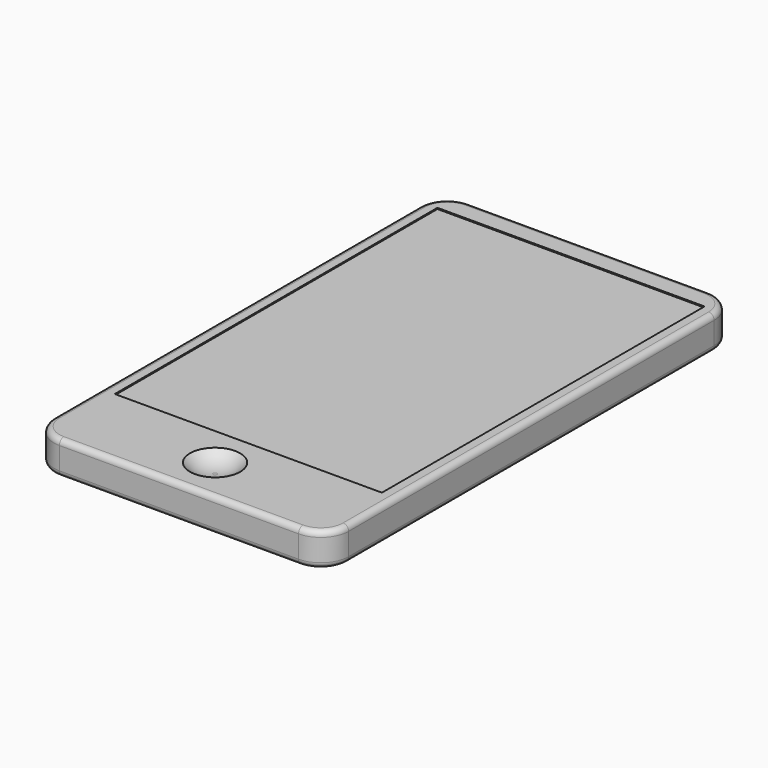
from build123d import *

# Parameters (mm, degrees)
F1_DEPTH  = 3.81
F2_R      = 1.27
F3_R      = 5.7323628205
F4_DEPTH  = 2.286
F3_W      = 60.96
F3_H      = 92.0373842978
F6_DEPTH  = 0.254
F7_W      = 12.1530219913
F7_H      = 2.4910259526
F8_DEPTH  = 1.1176
F9_R      = 0.9198153673
F11_DEPTH = 1.6002
F12_R     = 0.3066051224


# Not quite as in the source:
# - a fillet or chamfer that OpenCascade refuses, or shapes differently, is made with other operations: its cross-section is extruded or revolved along the edge and cut away or added


with BuildPart() as f1:
    # F0 (on Top) → F1 (new body, symmetric)
    with BuildSketch(Plane.XY):
        with BuildLine():
            Line((-27.2898482323, -58.4841631353), (27.2898482323, -58.4841631353))
            ThreePointArc((27.2898482323, -58.4841631353), (31.7799762928, -56.6242911958), (33.6398482323, -52.1341631353))
            Line((33.6398482323, -52.1341631353), (33.6398482323, 52.1341631353))
            ThreePointArc((33.6398482323, 52.1341631353), (31.7799762928, 56.6242911958), (27.2898482323, 58.4841631353))
            Line((27.2898482323, 58.4841631353), (-27.2898482323, 58.4841631353))
            ThreePointArc((-27.2898482323, 58.4841631353), (-31.7799762928, 56.6242911958), (-33.6398482323, 52.1341631353))
            Line((-33.6398482323, 52.1341631353), (-33.6398482323, -52.1341631353))
            ThreePointArc((-33.6398482323, -52.1341631353), (-31.7799762928, -56.6242911958), (-27.2898482323, -58.4841631353))
        make_face()
    extrude(amount=F1_DEPTH, both=True)

    # F2
    f2_edges = [f1.edges().sort_by_distance(p)[0] for p in [
        (33.639848, 0, 3.81),
        (33.639848, 0, -3.81),
        (-33.639848, 0, -3.81),
        (-33.639848, 0, 3.81),
        (-31.779976, 56.624291, -3.81),
        (-31.779976, 56.624291, 3.81),
        (0, 58.484163, -3.81),
        (0, 58.484163, 3.81),
        (31.779976, 56.624291, -3.81),
        (31.779976, 56.624291, 3.81),
        (31.779976, -56.624291, -3.81),
        (31.779976, -56.624291, 3.81),
        (0, -58.484163, -3.81),
        (0, -58.484163, 3.81),
        (-31.779976, -56.624291, 3.81),
        (-31.779976, -56.624291, -3.81),
    ]]
    fillet(f2_edges, radius=F2_R)

    # F3 (on face) → F4 (cut)
    with BuildSketch(Plane.XY.offset(3.81)):
        with Locations((0, -48.1907315552)):
            Circle(F3_R)
    extrude(amount=-F4_DEPTH, mode=Mode.SUBTRACT)

    # F5: fillet of radius 7.2972019136 on 1 edges, made by hand

    # F5_s1 → F5_t2 (revolve)
    with BuildSketch(Plane.XZ.offset(48.1907315552)):
        with BuildLine():
            ThreePointArc((5.7323628205, 3.81), (3.3159569781, 2.1198248924), (0.4279296605, 1.524))
            Line((0.4279296605, 1.524), (5.7323628205, 1.524))
            Line((5.7323628205, 1.524), (5.7323628205, 3.81))
        make_face()
    revolve(axis=Axis((0, -48.1907315552, 1.524), (0, 0, 1)))

    # F3 (on face) → F6 (cut)
    with BuildSketch(Plane.XY.offset(3.81)):
        with Locations((0, 7.3213078511)):
            Rectangle(F3_W, F3_H)
    extrude(amount=-F6_DEPTH, mode=Mode.SUBTRACT)

    # F7 (on face) → F8 (cut)
    with BuildSketch(Plane(origin=(-33.6398482323, 0, 0), x_dir=(0, -1, 0), z_dir=(-1, 0, 0))):
        with Locations((-43.15578565, 0)):
            Rectangle(F7_W, F7_H)
    extrude(amount=-F8_DEPTH, mode=Mode.SUBTRACT)

    # F9
    f9_edges = [f1.edges().sort_by_distance(p)[0] for p in [
        (-33.081048, 37.079275, 1.245513),
        (-33.081048, 49.232297, 1.245513),
        (-33.081048, 49.232297, -1.245513),
        (-33.081048, 37.079275, -1.245513),
    ]]
    fillet(f9_edges, radius=F9_R)


with BuildPart() as f11:
    # F10 (on face) → F11 (new body)
    with BuildSketch(Plane(origin=(-32.5222482323, 0, 0), x_dir=(0, -1, 0), z_dir=(-1, 0, 0))):
        with BuildLine():
            Line((-48.3124812784, -1.0677123209), (-37.9990900217, -1.0677123209))
            ThreePointArc((-37.9990900217, -1.0677123209), (-37.4744063871, -0.8503812436), (-37.2570753098, -0.325697609))
            Line((-37.2570753098, -0.325697609), (-37.2570753098, 0.325697609))
            ThreePointArc((-37.2570753098, 0.325697609), (-37.4744063871, 0.8503812436), (-37.9990900217, 1.0677123209))
            Line((-37.9990900217, 1.0677123209), (-48.3124812784, 1.0677123209))
            ThreePointArc((-48.3124812784, 1.0677123209), (-48.8371649129, 0.8503812436), (-49.0544959903, 0.325697609))
            Line((-49.0544959903, 0.325697609), (-49.0544959903, -0.325697609))
            ThreePointArc((-49.0544959903, -0.325697609), (-48.8371649129, -0.8503812436), (-48.3124812784, -1.0677123209))
        make_face()
    extrude(amount=F11_DEPTH)

    # F12
    f12_edges = [f11.edges().sort_by_distance(p)[0] for p in [
        (-34.122448, 37.474406, -0.850381),
        (-34.122448, 37.257075, 0),
        (-34.122448, 37.474406, 0.850381),
        (-34.122448, 43.155786, 1.067712),
        (-34.122448, 48.837165, 0.850381),
        (-34.122448, 49.054496, 0),
        (-34.122448, 48.837165, -0.850381),
        (-34.122448, 43.155786, -1.067712),
    ]]
    fillet(f12_edges, radius=F12_R)


solid = Compound([f1.part, f11.part])
